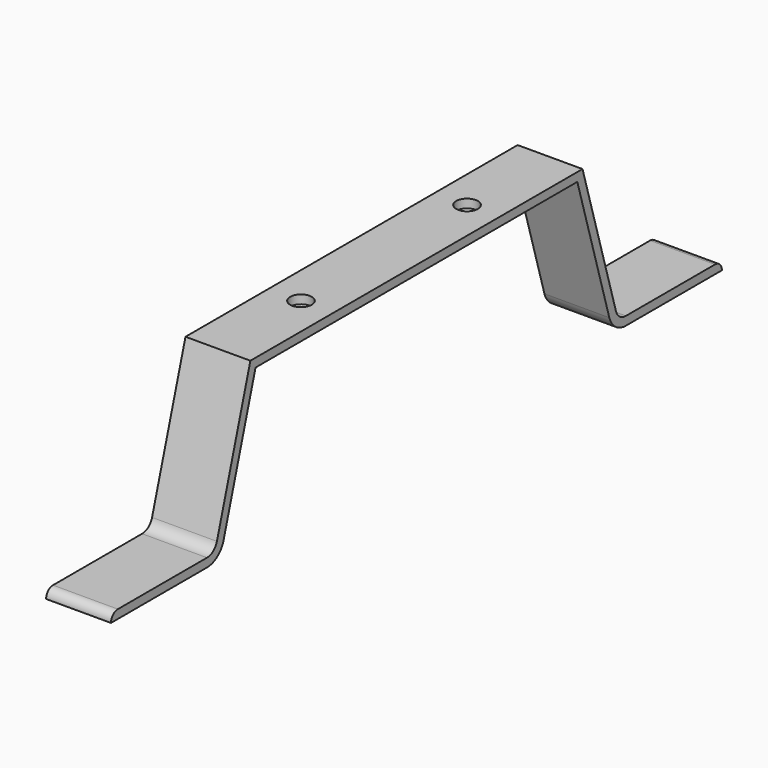
from build123d import *

# Parameters (mm, degrees)
F1_DEPTH = 7.5
F2_R     = 2.5
F3_DEPTH = 2
F4_R     = 5
F5_R     = 3
F6_R     = 3
F7_R     = 5
F8_R     = 1.999


# Not quite as in the source:
# - a fillet or chamfer is up to 0.001 mm smaller than in the source, because OpenCascade refuses the exact size


with BuildPart() as f1:
    # F0 (on Right) → F1 (new body, symmetric)
    with BuildSketch(Plane.YZ):
        Polygon((-58.3, 0), (-88.3, 0), (-88.2997653641, -2), (-56.8037653641, -2), (-46.5037653641, 33), (0, 33), (46.5037653641, 33), (56.8037653641, -2), (88.2997653641, -2), (88.3, 0), (58.3, 0), (48, 35), (0, 35), (-48, 35), align=None)
    extrude(amount=F1_DEPTH, both=True)

    # F2 (on face) → F3 (cut)
    with BuildSketch(Plane.XY.offset(35)):
        with Locations((0, -24)):
            Circle(F2_R)
        with Locations((0, 24)):
            Circle(F2_R)
    extrude(amount=-F3_DEPTH, mode=Mode.SUBTRACT)

    # F4
    f4_edges = [f1.edges().sort_by_distance(p)[0] for p in [
        (0, -56.803765, -2),
    ]]
    fillet(f4_edges, radius=F4_R)

    # F5
    f5_edges = [f1.edges().sort_by_distance(p)[0] for p in [
        (0, -58.3, 0),
    ]]
    fillet(f5_edges, radius=F5_R)

    # F6
    f6_edges = [f1.edges().sort_by_distance(p)[0] for p in [
        (0, 58.3, 0),
    ]]
    fillet(f6_edges, radius=F6_R)

    # F7
    f7_edges = [f1.edges().sort_by_distance(p)[0] for p in [
        (0, 56.803765, -2),
    ]]
    fillet(f7_edges, radius=F7_R)

    # F8 (radius 2 in the source; OpenCascade refuses exactly that, so slightly less here)
    f8_edges = [f1.edges().sort_by_distance(p)[0] for p in [
        (0, -88.3, 0),
        (0, 88.3, 0),
    ]]
    fillet(f8_edges, radius=F8_R)


solid = f1.part
